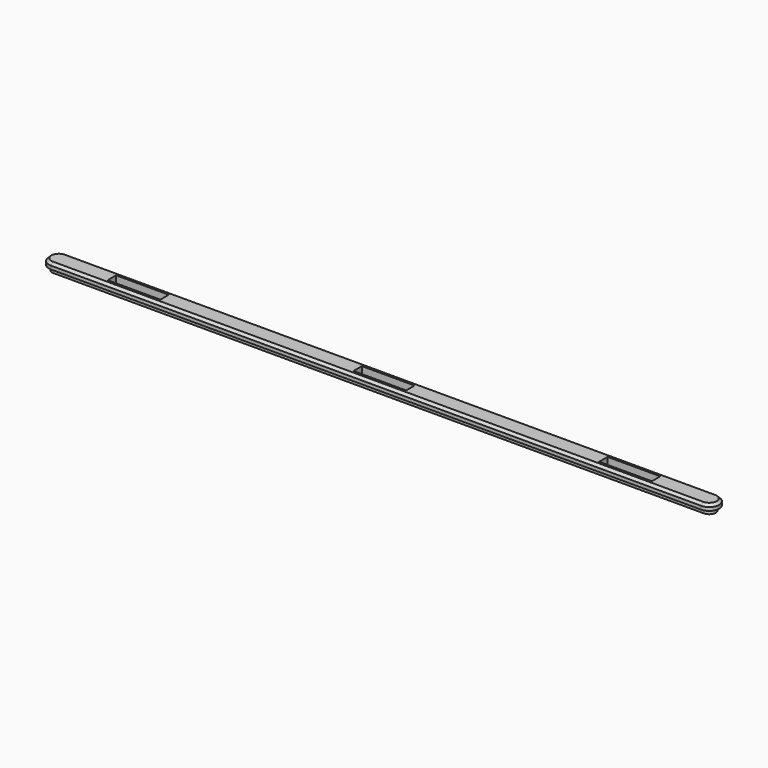
from build123d import *

# Parameters (mm, degrees)
F0_W          = 200
F0_H          = 4
F1_DEPTH      = 1.4
F2_R          = 1.99999
F5_DEPTH      = 1.775
F6_SIZE       = 0.75
F7_DEPTH      = 1.4
F7_DEPTH_BACK = 25


# Not quite as in the source:
# - a fillet or chamfer is up to 0.001 mm smaller than in the source, because OpenCascade refuses the exact size


with BuildPart() as f1:
    # F0 (on Top) → F1 (new body)
    with BuildSketch(Plane.XY):
        with Locations((100, 2)):
            Rectangle(F0_W, F0_H)
    extrude(amount=F1_DEPTH)

    # F2 (radius 2 in the source; OpenCascade refuses exactly that, so slightly less here)
    f2_edges = [f1.edges().sort_by_distance(p)[0] for p in [
        (0, 0, 0.7),
        (0, 4, 0.7),
        (200, 0, 0.7),
        (200, 4, 0.7),
    ]]
    fillet(f2_edges, radius=F2_R)

    # F4 (on face) → F5 (join)
    with BuildSketch(Plane.XY.offset(1.4)):
        with BuildLine():
            Line((198, 5), (2, 5))
            ThreePointArc((2, 5), (-1, 2), (2, -1))
            Line((2, -1), (198, -1))
            ThreePointArc((198, -1), (201, 2), (198, 5))
        make_face()
    extrude(amount=F5_DEPTH)

    # F6
    f6_edges = [f1.edges().sort_by_distance(p)[0] for p in [
        (-1, 2, 3.175),
    ]]
    chamfer(f6_edges, length=F6_SIZE)

    # F3 (on face) → F7 (cut, two sides)
    with BuildSketch(Plane.XY.offset(1.4)) as f7_sk:
        Polygon((18, 3.5875), (18, 2), (18, 0.4125), (33.875, 0.4125), (33.875, 3.5875), align=None)
        Polygon((182, 0.4125), (182, 2), (182, 3.5875), (166.125, 3.5875), (166.125, 0.4125), align=None)
        Polygon((92.0625, 3.5875), (92.0625, 2), (92.0625, 0.4125), (107.9375, 0.4125), (107.9375, 3.5875), align=None)
    extrude(amount=-F7_DEPTH, mode=Mode.SUBTRACT)
    extrude(f7_sk.sketch, amount=F7_DEPTH_BACK, mode=Mode.SUBTRACT)


solid = f1.part
